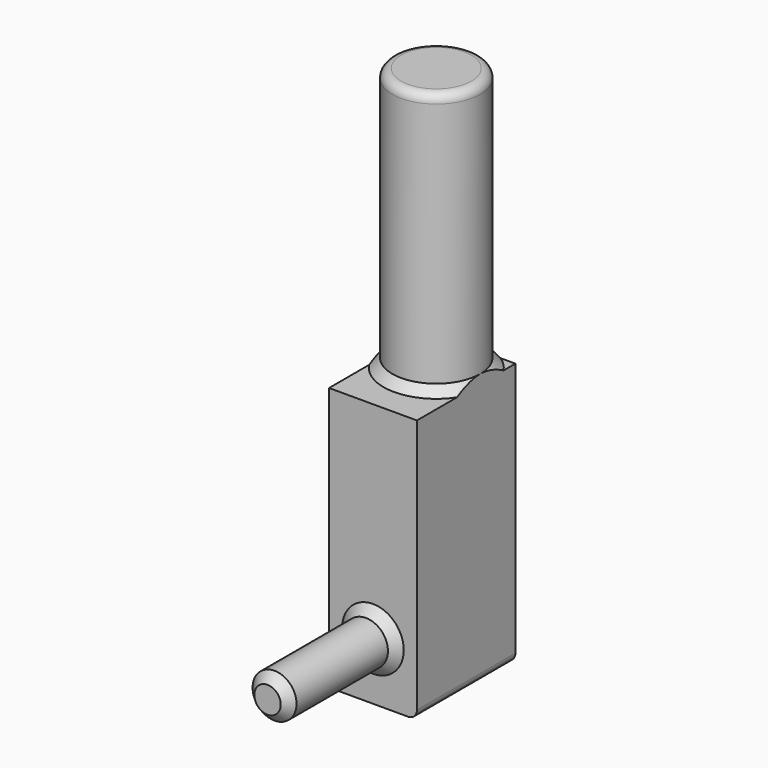
from build123d import *

# Parameters (mm, degrees)
F1_W         = 70
F1_H         = 150
F2_DEPTH     = 25
F0_R         = 25
F3_DEPTH     = 150
F4_R         = 5
F5_R         = 5
F6_R         = 5
F7_T4_ANGLE  = 180
F7_T10_ANGLE = 90
F7_T16_ANGLE = 90
F8_R         = 12.5
F9_DEPTH     = 120
F10_SIZE     = 5


# Not quite as in the source:
# - a fillet or chamfer that OpenCascade refuses, or shapes differently, is made with other operations: its cross-section is extruded or revolved along the edge and cut away or added


with BuildPart() as f2:
    # F1 (on Right) → F2 (new body, symmetric)
    with BuildSketch(Plane.YZ):
        with Locations((-10, -75)):
            Rectangle(F1_W, F1_H)
    extrude(amount=F2_DEPTH, both=True)

    # F0 (on Top) → F3 (join)
    with BuildSketch(Plane.XY):
        Circle(F0_R)
    extrude(amount=F3_DEPTH)

    # F4
    f4_edges = [f2.edges().sort_by_distance(p)[0] for p in [
        (-25, 0, 150),
    ]]
    fillet(f4_edges, radius=F4_R)

    # F5
    f5_edges = [f2.edges().sort_by_distance(p)[0] for p in [
        (-25, -10, -150),
    ]]
    fillet(f5_edges, radius=F5_R)

    # F6
    f6_edges = [f2.edges().sort_by_distance(p)[0] for p in [
        (25, -10, -150),
    ]]
    fillet(f6_edges, radius=F6_R)

    # F7: chamfer of 5 on 3 edges, made by hand


with BuildPart() as f7_tool2:
    # F7_s3 → F7_t4 (revolve)
    with BuildSketch(Plane.XZ):
        Polygon((-30, 0), (-25, 5), (-25, 0), align=None)
    revolve(axis=Axis((0, 0, 0), (0, 0, 1)), revolution_arc=F7_T4_ANGLE)

    split(bisect_by=Plane.YZ.offset(25), keep=Keep.BOTTOM)

    split(bisect_by=Plane.YZ.offset(-25), keep=Keep.TOP)


with BuildPart() as f2_1:
    add(f2.part)

    # F7_t1: union F7_tool2
    add(f7_tool2.part)


with BuildPart() as f7_tool8:
    # F7_s9 → F7_t10 (revolve)
    with BuildSketch(Plane.XZ):
        Polygon((30, 0), (25, 5), (25, 0), align=None)
    revolve(axis=Axis((0, 0, 0), (0, 0, 1)), revolution_arc=F7_T10_ANGLE)

    split(bisect_by=Plane.YZ.offset(25), keep=Keep.BOTTOM)

    split(bisect_by=Plane.XZ.offset(-25), keep=Keep.TOP)


with BuildPart() as f2_2:
    add(f2_1.part)

    # F7_t7: union F7_tool8
    add(f7_tool8.part)


with BuildPart() as f7_tool14:
    # F7_s15 → F7_t16 (revolve)
    with BuildSketch(Plane.YZ):
        Polygon((30, 0), (25, 5), (25, 0), align=None)
    revolve(axis=Axis((0, 0, 0), (0, 0, 1)), revolution_arc=F7_T16_ANGLE)

    split(bisect_by=Plane.YZ.offset(-25), keep=Keep.TOP)

    split(bisect_by=Plane.XZ.offset(-25), keep=Keep.TOP)


with BuildPart() as f2_3:
    add(f2_2.part)

    # F7_t13: union F7_tool14
    add(f7_tool14.part)

    # F8 (on Front) → F9 (join)
    with BuildSketch(Plane.XZ):
        with Locations((0, -117.5)):
            Circle(F8_R)
    extrude(amount=F9_DEPTH)

    # F10
    f10_edges = [f2_3.edges().sort_by_distance(p)[0] for p in [
        (-12.5, -120, -117.5),
        (-12.5, -45, -117.5),
    ]]
    chamfer(f10_edges, length=F10_SIZE)


solid = f2_3.part
